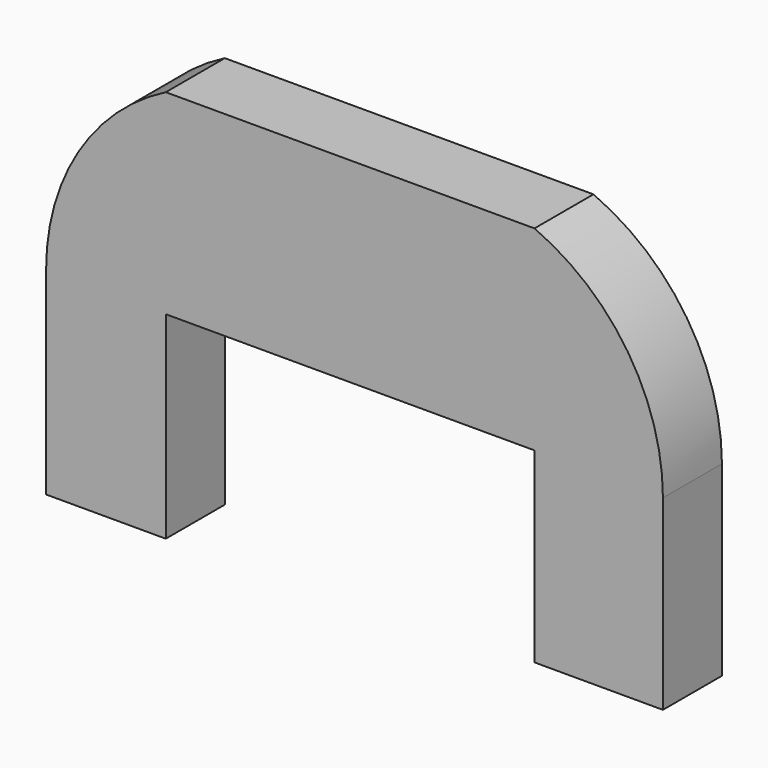
from build123d import *

# Parameters (mm, degrees)
F0_W     = 127
F0_H     = 67.3248254269
F0_W_2   = 44.2579090595
F0_H_2   = 64.2999485135
F0_W_3   = 41.2393848896
F0_H_3   = 68.0945366621
F1_DEPTH = 25.4


with BuildPart() as f1:
    # F0 (on Front) → F1 (new body)
    with BuildSketch(Plane.XZ):
        with Locations((-63.5, 33.6624127134)):
            Rectangle(F0_W, F0_H)
        with BuildLine():
            Line((0, 67.3248254269), (0, 0))
            Line((0, 0), (44.2579090595, 0))
            ThreePointArc((44.2579090595, 0), (32.2025736705, 40.2845957938), (0, 67.3248254269))
        make_face()
        with Locations((22.1289545298, -32.1499742568)):
            Rectangle(F0_W_2, F0_H_2)
        with BuildLine():
            Line((-168.2393848896, 0), (-127, 0))
            Line((-127, 0), (-127, 67.3248254269))
            ThreePointArc((-127, 67.3248254269), (-157.1100758974, 39.4756855065), (-168.2393848896, 0))
        make_face()
        with Locations((-147.6196924448, -34.0472683311)):
            Rectangle(F0_W_3, F0_H_3)
    extrude(amount=F1_DEPTH)


solid = f1.part
